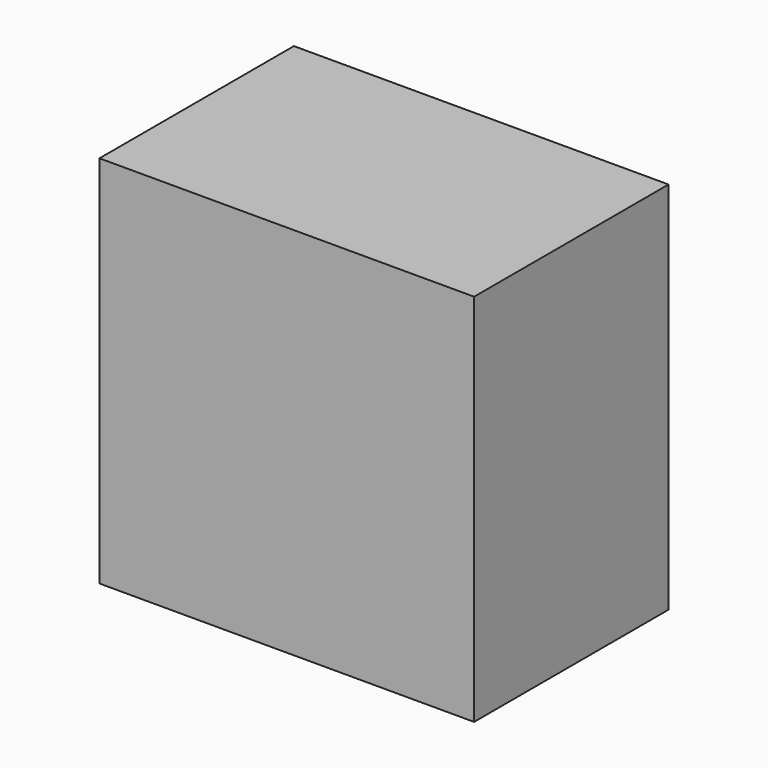
from build123d import *

# Parameters (mm, degrees)
F2_W     = 46.9865724444
F2_H     = 46.9472724944
F3_DEPTH = 30.48


# Not quite as in the source:
# - the program builds the solid bodies; features that only make, move or delete a surface that nothing else refers to are left out


with BuildPart() as f3:
    # F2 (on Front) → F3 (new body)
    with BuildSketch(Plane.XZ):
        with Locations((-95.4283364117, -43.9801728353)):
            Rectangle(F2_W, F2_H)
    extrude(amount=F3_DEPTH)


solid = f3.part
